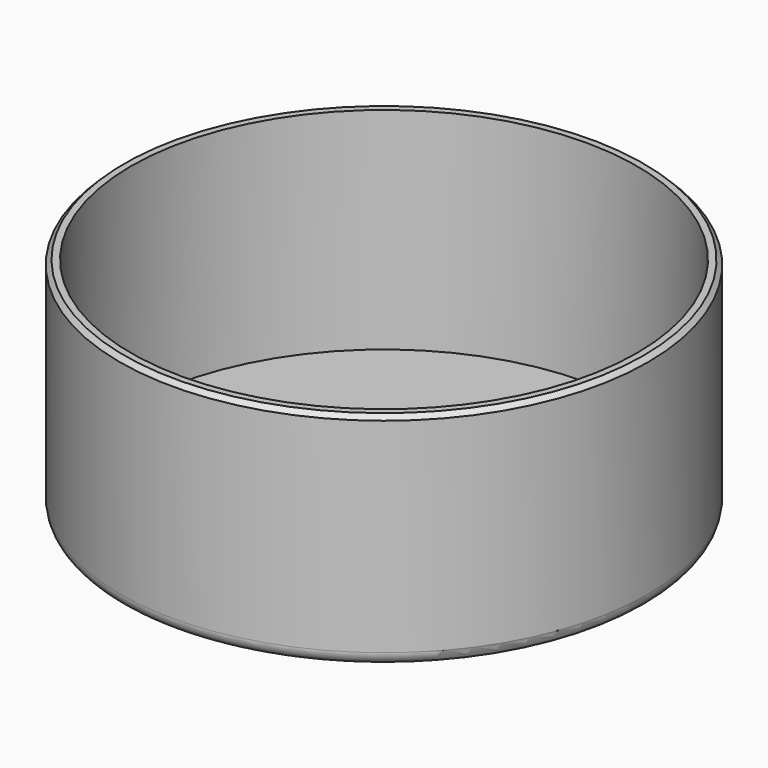
from build123d import *

# Parameters (mm, degrees)
F0_R           = 59.5
F1_DEPTH       = 50
F2_T           = -2.5
F3_R           = 3
F4_R           = 44.5
F4_TEXT_SIZE   = 29.2763178651
F4_TEXT_SIZE_2 = 28.2475105719
F4_TEXT_SIZE_3 = 27.6315789152
F5_DEPTH       = 2.2
F6_SIZE        = 1


# Not quite as in the source:
# - Text() gives the source's letters only with a copy of the font that has no kerning and outlines rounded to 1/6400 em; it was checked with that copy


with BuildPart() as f1:
    # F0 (on Top) → F1 (new body)
    with BuildSketch(Plane.XY):
        Circle(F0_R)
    extrude(amount=F1_DEPTH)

    # F2
    f2_openings = [f1.faces().sort_by_distance(p)[0] for p in [
        (0, 0, 50),
    ]]
    offset(amount=F2_T, openings=f2_openings)

    # F3
    f3_edges = [f1.edges().sort_by_distance(p)[0] for p in [
        (-59.5, 0, 0),
    ]]
    fillet(f3_edges, radius=F3_R)

    # F4 (on face) → F5 (cut)
    with BuildSketch(Plane(origin=(0, 0, 0), x_dir=(1, 0, 0), z_dir=(0, 0, -1))):
        Circle(F4_R)
        with BuildLine():
            ThreePointArc((37.2958897161, 20.3780914289), (41.1784246477, 10.5160517084), (42.5, 0))
            ThreePointArc((42.5, 0), (30.4035359786, -29.6963802508), (1, -42.4882336653))
            ThreePointArc((1, -42.4882336653), (0, -42.5), (-1, -42.4882336653))
            ThreePointArc((-1, -42.4882336653), (-36.8060796608, -21.25), (-37.2958897161, 20.3780914289))
            ThreePointArc((-37.2958897161, 20.3780914289), (-36.8060796608, 21.25), (-36.2958897161, 22.1101422365))
            ThreePointArc((-36.2958897161, 22.1101422365), (0, 42.5), (36.2958897161, 22.1101422365))
            ThreePointArc((36.2958897161, 22.1101422365), (36.8060796608, 21.25), (37.2958897161, 20.3780914289))
        make_face(mode=Mode.SUBTRACT)
        with BuildLine():
            Line((1, -0.5773502692), (37.2958897161, 20.3780914289))
            ThreePointArc((37.2958897161, 20.3780914289), (36.8060796608, 21.25), (36.2958897161, 22.1101422365))
            Line((36.2958897161, 22.1101422365), (0, 1.1547005384))
            Line((0, 1.1547005384), (-36.2958897161, 22.1101422365))
            ThreePointArc((-36.2958897161, 22.1101422365), (-36.8060796608, 21.25), (-37.2958897161, 20.3780914289))
            Line((-37.2958897161, 20.3780914289), (-1, -0.5773502692))
            Line((-1, -0.5773502692), (-1, -42.4882336653))
            ThreePointArc((-1, -42.4882336653), (0, -42.5), (1, -42.4882336653))
            Line((1, -42.4882336653), (1, -0.5773502692))
        make_face()
        with Locations((-30.4032191634, -22.3971046507)):
            Text('P', F4_TEXT_SIZE, font='Open Sans', text_align=(TextAlign.LEFT, TextAlign.BOTTOM))
        with Locations((-12.2876670988, 13.2635878399)):
            Text('M', F4_TEXT_SIZE_2, font='Open Sans', text_align=(TextAlign.LEFT, TextAlign.BOTTOM))
        with Locations((10.0967809558, -21.2128926069)):
            Text('O', F4_TEXT_SIZE_3, font='Open Sans', text_align=(TextAlign.LEFT, TextAlign.BOTTOM))
    extrude(amount=-F5_DEPTH, mode=Mode.SUBTRACT)

    # F6
    f6_edges = [f1.edges().sort_by_distance(p)[0] for p in [
        (-59.5, 0, 50),
    ]]
    chamfer(f6_edges, length=F6_SIZE)


solid = f1.part
